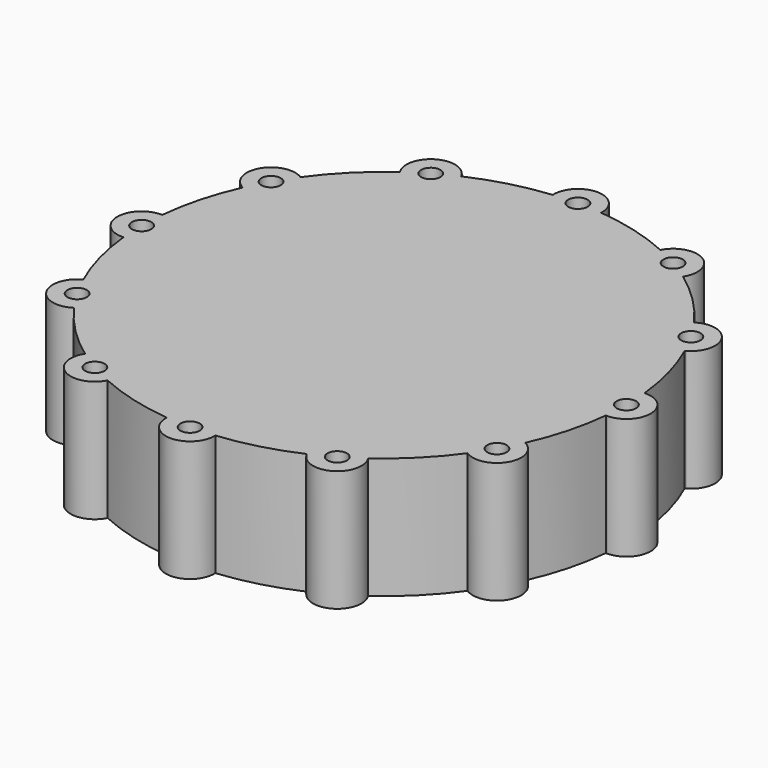
from build123d import *

# Parameters (mm, degrees)
F1_DEPTH = 25
F2_COUNT = 12
F3_R     = 40
F4_DEPTH = 10
F5_R     = 9.99999
F7_D     = 4


# Not quite as in the source:
# - a fillet or chamfer is up to 0.001 mm smaller than in the source, because OpenCascade refuses the exact size


with BuildPart() as f1:
    # F0 (on Top) → F1 (new body)
    with BuildSketch(Plane.XY):
        with BuildLine():
            ThreePointArc((-4.9937460889, 49.75), (-33.5433502766, -37.0788841825), (50, 0))
            ThreePointArc((50, 0), (37.0788841825, 33.5433502766), (4.9937460889, 49.75))
            ThreePointArc((4.9937460889, 49.75), (0, 45), (-4.9937460889, 49.75))
        make_face()
        with BuildLine():
            ThreePointArc((-4.9937460889, 49.75), (0, 45), (4.9937460889, 49.75))
            ThreePointArc((4.9937460889, 49.75), (0, 50), (-4.9937460889, 49.75))
        make_face()
        with BuildLine():
            ThreePointArc((-4.9937460889, 49.75), (0, 50), (4.9937460889, 49.75))
            ThreePointArc((4.9937460889, 49.75), (4.9984362777, 49.8749608947), (5, 50))
            ThreePointArc((5, 50), (-0.1250391053, 54.9984362777), (-4.9937460889, 49.75))
        make_face()
    extrude(amount=F1_DEPTH)

    # F2: F1 ×12 about axis
    f2_axis = Axis((0, 0, 0), (0, 0, -1))


with BuildPart() as f1_1:
    add(f1.part)
    for i in range(1, F2_COUNT):
        add(f1.part.rotate(f2_axis, i * 360 / F2_COUNT))

    # F3 (on face) → F4 (cut)
    with BuildSketch(Plane(origin=(0, 0, 0), x_dir=(1, 0, 0), z_dir=(0, 0, -1))):
        Circle(F3_R)
    extrude(amount=-F4_DEPTH, mode=Mode.SUBTRACT)

    # F5 (radius 10 in the source; OpenCascade refuses exactly that, so slightly less here)
    f5_edges = [f1_1.edges().sort_by_distance(p)[0] for p in [
        (-40, 0, 10),
    ]]
    fillet(f5_edges, radius=F5_R)

    # F7 (through all)
    with Locations(Plane.XY.offset(25)):
        with Locations((25, 43.3012701892), (43.3012701892, 25), (50, 0), (43.3012701892, -25), (25, -43.3012701892), (0, -50), (-25, -43.3012701892), (-43.3012701892, -25), (-50, 0), (-43.3012701892, 25), (-25, 43.3012701892), (0, 50)):
            Hole(F7_D / 2)


solid = f1_1.part
